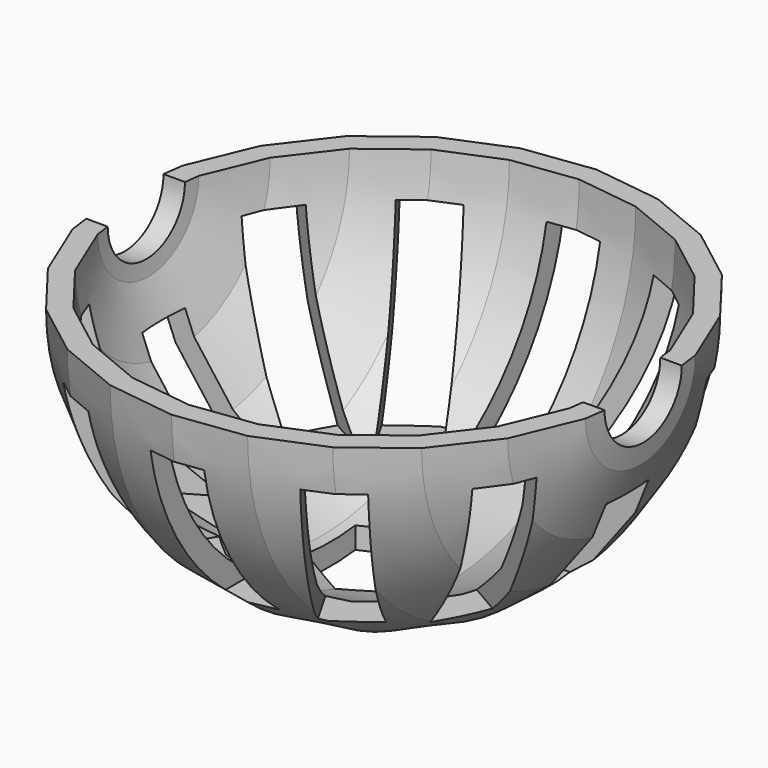
from build123d import *

# Parameters (mm, degrees)
F3_W           = 49.9716736376
F3_H           = 50
F4_DEPTH       = 25
F8_START       = 5
F7_W           = 55
F7_H           = 55
F8_DEPTH       = 20
F11_R          = 4.5
F12_DEPTH      = 25
F12_DEPTH_BACK = 25
F20_W          = 5
F20_H          = 15
F21_DEPTH      = 25
F21_DEPTH_BACK = 25
F22_W          = 5
F22_H          = 15
F23_DEPTH      = 25
F23_DEPTH_BACK = 25
F24_W          = 5
F24_H          = 15
F25_DEPTH      = 25
F25_DEPTH_BACK = 25
F26_W          = 5
F26_H          = 15
F27_DEPTH      = 25
F27_DEPTH_BACK = 25
F28_W          = 5
F28_H          = 15
F29_DEPTH      = 25
F29_DEPTH_BACK = 25
F30_W          = 5
F30_H          = 10
F31_DEPTH      = 25
F31_DEPTH_BACK = 25
F33_DEPTH      = 25
F33_DEPTH_BACK = 25


# Not quite as in the source:
# - a feature of the source that left no trace in its solid (it failed there, or was rolled back) is left out


with BuildPart() as f2:
    # F1 (on Top) → F2 (revolve)
    with BuildSketch(Plane.XY):
        Polygon((-22.74, 0), (-24.74, 0), (-23.8970049424, -6.4031831758), (-21.4254684896, -12.37), (-17.4938217666, -17.4938217666), (-12.37, -21.4254684896), (-6.4031831758, -23.8970049424), (0, -24.74), (6.4031831758, -23.8970049424), (12.37, -21.4254684896), (17.4938217666, -17.4938217666), (21.4254684896, -12.37), (23.8970049424, -6.4031831758), (24.74, 0), (22.74, 0), (21.9651532898, -5.8855450856), (19.6934176821, -11.37), (16.0796082042, -16.0796082042), (11.37, -19.6934176821), (5.8855450856, -21.9651532898), (0, -22.74), (-5.8855450856, -21.9651532898), (-11.37, -19.6934176821), (-16.0796082042, -16.0796082042), (-19.6934176821, -11.37), (-21.9651532898, -5.8855450856), align=None)
    revolve(axis=Axis((0, 0, 0), (1, 0, 0)))

    # F3 (on Top) → F4 (cut)
    with BuildSketch(Plane.XY):
        Rectangle(F3_W, F3_H)
    extrude(amount=F4_DEPTH, mode=Mode.SUBTRACT)


with BuildPart() as f6:
    # F5 (on Top) → F6 (revolve)
    with BuildSketch(Plane.XY):
        Polygon((-20.74, 0), (-22.74, 0), (-21.9651532898, -5.8855450856), (-19.6934176821, -11.37), (-16.0796082042, -16.0796082042), (-11.37, -19.6934176821), (-5.8855450856, -21.9651532898), (0, -22.74), (5.8855450856, -21.9651532898), (11.37, -19.6934176821), (16.0796082042, -16.0796082042), (19.6934176821, -11.37), (21.9651532898, -5.8855450856), (22.74, 0), (20.74, 0), (20.0333016372, -5.3679069954), (17.9613668745, -10.37), (14.6653946418, -14.6653946418), (10.37, -17.9613668745), (5.3679069954, -20.0333016372), (0, -20.74), (-5.3679069954, -20.0333016372), (-10.37, -17.9613668745), (-14.6653946418, -14.6653946418), (-17.9613668745, -10.37), (-20.0333016372, -5.3679069954), align=None)
    revolve(axis=Axis((0, 0, 0), (1, 0, 0)))

    # F7 (on Top) → F8 (cut)
    with BuildSketch(Plane.XY.offset(F8_START)):
        Rectangle(F7_W, F7_H)
    extrude(amount=F8_DEPTH, mode=Mode.SUBTRACT)


with BuildPart() as f12_tool:
    # F11 (on Right) → F12 (new body, two sides)
    with BuildSketch(Plane.YZ) as f12_sk:
        Circle(F11_R)
    extrude(amount=F12_DEPTH)
    extrude(f12_sk.sketch, amount=-F12_DEPTH_BACK)


with BuildPart() as f2_1:
    add(f2.part)

    # F12: cut by f12_tool
    add(f12_tool.part, mode=Mode.SUBTRACT)


with BuildPart() as f6_1:
    add(f6.part)

    # F12: cut by f12_tool
    add(f12_tool.part, mode=Mode.SUBTRACT)


with BuildPart() as f21_tool:
    # F20 (on Front) → F21 (new body, two sides)
    with BuildSketch(Plane.XZ) as f21_sk:
        with Locations((0, -11.5)):
            Rectangle(F20_W, F20_H)
    extrude(amount=-F21_DEPTH)
    extrude(f21_sk.sketch, amount=F21_DEPTH_BACK)


with BuildPart() as f2_2:
    add(f2_1.part)

    # F21: cut by f21_tool
    add(f21_tool.part, mode=Mode.SUBTRACT)


with BuildPart() as f6_2:
    add(f6_1.part)

    # F21: cut by f21_tool
    add(f21_tool.part, mode=Mode.SUBTRACT)


with BuildPart() as f23_tool:
    # F22 (on 3pt) → F23 (new body, two sides)
    with BuildSketch(Plane(origin=(0, 0, 0), x_dir=(0.8660254038, -0.5, 0), z_dir=(-0.5, -0.8660254038, 0))) as f23_sk:
        with Locations((0, -11.5)):
            Rectangle(F22_W, F22_H)
    extrude(amount=F23_DEPTH)
    extrude(f23_sk.sketch, amount=-F23_DEPTH_BACK)


with BuildPart() as f2_3:
    add(f2_2.part)

    # F23: cut by f23_tool
    add(f23_tool.part, mode=Mode.SUBTRACT)


with BuildPart() as f6_3:
    add(f6_2.part)

    # F23: cut by f23_tool
    add(f23_tool.part, mode=Mode.SUBTRACT)


with BuildPart() as f25_tool:
    # F24 (on 3pt) → F25 (new body, two sides)
    with BuildSketch(Plane(origin=(0, 0, 0), x_dir=(0.5, -0.8660254038, 0), z_dir=(-0.8660254038, -0.5, 0))) as f25_sk:
        with Locations((0, -11.5)):
            Rectangle(F24_W, F24_H)
    extrude(amount=-F25_DEPTH)
    extrude(f25_sk.sketch, amount=F25_DEPTH_BACK)


with BuildPart() as f2_4:
    add(f2_3.part)

    # F25: cut by f25_tool
    add(f25_tool.part, mode=Mode.SUBTRACT)


with BuildPart() as f6_4:
    add(f6_3.part)

    # F25: cut by f25_tool
    add(f25_tool.part, mode=Mode.SUBTRACT)


with BuildPart() as f27_tool:
    # F26 (on 3pt) → F27 (new body, two sides)
    with BuildSketch(Plane(origin=(0, 0, 0), x_dir=(0.8660254038, 0.5, 0), z_dir=(0.5, -0.8660254038, 0))) as f27_sk:
        with Locations((0, -11.5)):
            Rectangle(F26_W, F26_H)
    extrude(amount=-F27_DEPTH)
    extrude(f27_sk.sketch, amount=F27_DEPTH_BACK)


with BuildPart() as f2_5:
    add(f2_4.part)

    # F27: cut by f27_tool
    add(f27_tool.part, mode=Mode.SUBTRACT)


with BuildPart() as f6_5:
    add(f6_4.part)

    # F27: cut by f27_tool
    add(f27_tool.part, mode=Mode.SUBTRACT)


with BuildPart() as f29_tool:
    # F28 (on 3pt) → F29 (new body, two sides)
    with BuildSketch(Plane(origin=(0, 0, 0), x_dir=(-0.5, -0.8660254038, 0), z_dir=(-0.8660254038, 0.5, 0))) as f29_sk:
        with Locations((0, -11.5)):
            Rectangle(F28_W, F28_H)
    extrude(amount=F29_DEPTH)
    extrude(f29_sk.sketch, amount=-F29_DEPTH_BACK)


with BuildPart() as f2_6:
    add(f2_5.part)

    # F29: cut by f29_tool
    add(f29_tool.part, mode=Mode.SUBTRACT)


with BuildPart() as f6_6:
    add(f6_5.part)

    # F29: cut by f29_tool
    add(f29_tool.part, mode=Mode.SUBTRACT)


with BuildPart() as f31_tool:
    # F30 (on Right) → F31 (new body, two sides)
    with BuildSketch(Plane.YZ) as f31_sk:
        with Locations((0, -14)):
            Rectangle(F30_W, F30_H)
    extrude(amount=-F31_DEPTH)
    extrude(f31_sk.sketch, amount=F31_DEPTH_BACK)


with BuildPart() as f2_7:
    add(f2_6.part)

    # F31: cut by f31_tool
    add(f31_tool.part, mode=Mode.SUBTRACT)


with BuildPart() as f6_7:
    add(f6_6.part)

    # F31: cut by f31_tool
    add(f31_tool.part, mode=Mode.SUBTRACT)


with BuildPart() as f33_tool:
    # F32 (on Top) → F33 (new body, two sides)
    with BuildSketch(Plane.XY) as f33_sk:
        Polygon((-0.0097421482, 5.7154667633), (-4.9546104856, 2.8492964339), (-4.9448683374, -2.8661703294), (0.0097421482, -5.7154667633), (4.9546104856, -2.8492964339), (4.9448683374, 2.8661703294), align=None)
    extrude(amount=-F33_DEPTH)
    extrude(f33_sk.sketch, amount=F33_DEPTH_BACK)


with BuildPart() as f2_8:
    add(f2_7.part)

    # F33: cut by f33_tool
    add(f33_tool.part, mode=Mode.SUBTRACT)


with BuildPart() as f6_8:
    add(f6_7.part)

    # F33: cut by f33_tool
    add(f33_tool.part, mode=Mode.SUBTRACT)


solid = f2_8.part
